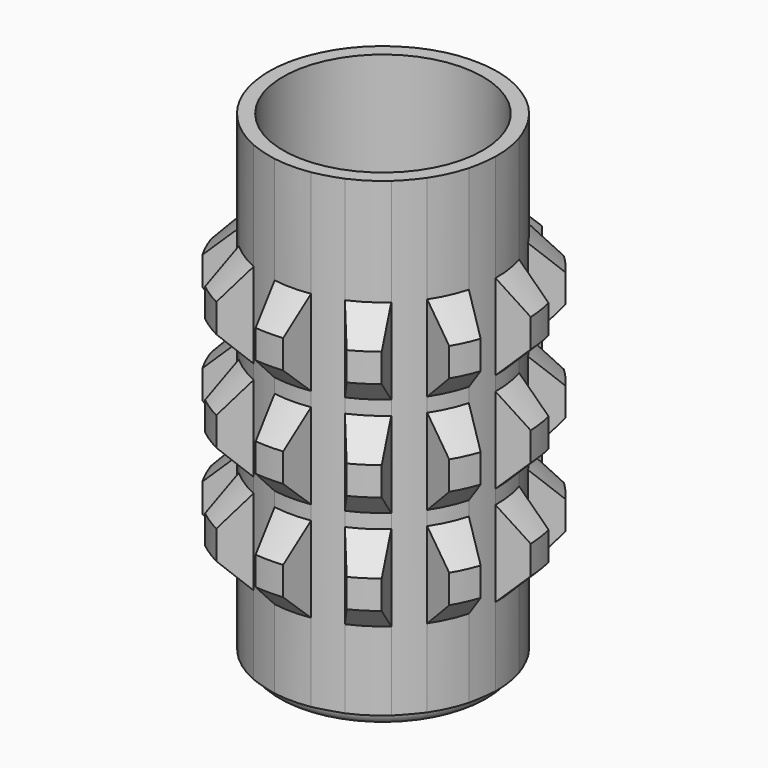
from build123d import *

# Parameters (mm, degrees)
F6_DEPTH = 225.001


# Not quite as in the source:
# - a feature names something its author has since deleted; it is built from what else it names


with BuildPart() as f1:
    # F0 (on Front) → F1 (revolve)
    with BuildSketch(Plane.XZ):
        with BuildLine():
            Line((40, -80), (40, 85))
            Line((40, 85), (35, 85))
            Line((35, 85), (35, -75))
            ThreePointArc((35, -75), (33.5355339059, -78.5355339059), (30, -80))
            Line((30, -80), (0, -80))
            Line((0, -80), (0, -85))
            Line((0, -85), (32.9289321881, -85))
            ThreePointArc((32.9289321881, -85), (37.5483298507, -81.9134171618), (36.4644660941, -76.4644660941))
            Line((36.4644660941, -76.4644660941), (40, -80))
        make_face()
    revolve(axis=Axis((0, 0, 2.5), (0, 0, 1)))

    # F2 (on Front) → F3 (revolve)
    with BuildSketch(Plane.XZ):
        Polygon((50, 37.5), (40, 47.5), (40, 17.5), (50, 27.5), align=None)
        Polygon((50, -7.5), (50, 2.5), (40, 12.5), (40, -17.5), align=None)
        Polygon((50, -42.5), (50, -32.5), (40, -22.5), (40, -52.5), align=None)
    revolve(axis=Axis((0, 0, 2.5), (0, 0, 1)))

    # F5 (on offset) → F6 (cut, through all)
    with BuildSketch(Plane.XY.offset(140)):
        with BuildLine():
            ThreePointArc((-18.8668219017, 48.0068175713), (-27.9042191508, 43.4198125328), (-35.8309761925, 37.104617598))
            Line((-35.8309761925, 37.104617598), (-25.6622849381, 30.6830104741))
            ThreePointArc((-25.6622849381, 30.6830104741), (-21.591517079, 33.5970563735), (-17.2497496098, 36.0894186487))
            Line((-17.2497496098, 36.0894186487), (-18.8668219017, 48.0068175713))
        make_face()
        with BuildLine():
            ThreePointArc((-5, 39.686269666), (0, 39.9368978106), (5, 39.686269666))
            Line((5, 39.686269666), (10.0826645171, 50.5860788976))
            ThreePointArc((10.0826645171, 50.5860788976), (0, 51.6132305402), (-10.0826645171, 50.5860788976))
            Line((-10.0826645171, 50.5860788976), (-5, 39.686269666))
        make_face()
        with BuildLine():
            ThreePointArc((-41.8262256733, 30.1857308662), (-46.949045883, 21.4409108359), (-50.2032060963, 11.8427023797))
            Line((-50.2032060963, 11.8427023797), (-38.1769757294, 11.9381122525))
            ThreePointArc((-38.1769757294, 11.9381122525), (-36.3278800438, 16.5903869233), (-34.0228255994, 21.0344322061))
            Line((-34.0228255994, 21.0344322061), (-41.8262256733, 30.1857308662))
        make_face()
        with BuildLine():
            ThreePointArc((-51.5060983236, 2.7808878932), (-51.0878822734, -7.3453285571), (-48.6362727834, -17.1791871675))
            Line((-48.6362727834, -17.1791871675), (-38.5707464723, -10.5970522586))
            ThreePointArc((-38.5707464723, -10.5970522586), (-39.5303977752, -5.6836131531), (-39.993894855, -0.6988378398))
            Line((-39.993894855, -0.6988378398), (-51.5060983236, 2.7808878932))
        make_face()
        with BuildLine():
            ThreePointArc((-44.8331486809, -25.5068673371), (-39.0066770118, -33.7994780328), (-31.6276665093, -40.7468061715))
            Line((-31.6276665093, -40.7468061715), (-26.718577738, -29.7677275528))
            ThreePointArc((-26.718577738, -29.7677275528), (-30.1822935214, -26.1531062118), (-33.2671850775, -22.2102318092))
            Line((-33.2671850775, -22.2102318092), (-44.8331486809, -25.5068673371))
        make_face()
        with BuildLine():
            ThreePointArc((-23.9259911079, -45.6963724108), (-14.5411274069, -49.5225320489), (-4.5774995889, -51.3776021191))
            Line((-4.5774995889, -51.3776021191), (-6.3834493564, -39.4873596777))
            ThreePointArc((-6.3834493564, -39.4873596777), (-11.2515243325, -38.3191728373), (-15.9783790926, -36.6700341093))
            Line((-15.9783790926, -36.6700341093), (-23.9259911079, -45.6963724108))
        make_face()
        with BuildLine():
            ThreePointArc((4.5774995889, -51.3776021191), (14.5411274069, -49.5225320489), (23.9259911079, -45.6963724108))
            Line((23.9259911079, -45.6963724108), (15.9783790926, -36.6700341093))
            ThreePointArc((15.9783790926, -36.6700341093), (11.2515243325, -38.3191728373), (6.3834493564, -39.4873596777))
            Line((6.3834493564, -39.4873596777), (4.5774995889, -51.3776021191))
        make_face()
        with BuildLine():
            ThreePointArc((31.6276665093, -40.7468061715), (39.0066770118, -33.7994780328), (44.8331486809, -25.5068673371))
            Line((44.8331486809, -25.5068673371), (33.2671850775, -22.2102318092))
            ThreePointArc((33.2671850775, -22.2102318092), (30.1822935214, -26.1531062118), (26.718577738, -29.7677275528))
            Line((26.718577738, -29.7677275528), (31.6276665093, -40.7468061715))
        make_face()
        with BuildLine():
            ThreePointArc((48.6362727834, -17.1791871675), (51.0878822734, -7.3453285571), (51.5060983236, 2.7808878932))
            Line((51.5060983236, 2.7808878932), (39.993894855, -0.6988378398))
            ThreePointArc((39.993894855, -0.6988378398), (39.5303977752, -5.6836131531), (38.5707464723, -10.5970522586))
            Line((38.5707464723, -10.5970522586), (48.6362727834, -17.1791871675))
        make_face()
        with BuildLine():
            ThreePointArc((50.2032060963, 11.8427023797), (46.949045883, 21.4409108359), (41.8262256733, 30.1857308662))
            Line((41.8262256733, 30.1857308662), (34.0228255994, 21.0344322061))
            ThreePointArc((34.0228255994, 21.0344322061), (36.3278800438, 16.5903869233), (38.1769757294, 11.9381122525))
            Line((38.1769757294, 11.9381122525), (50.2032060963, 11.8427023797))
        make_face()
        with BuildLine():
            ThreePointArc((35.8309761925, 37.104617598), (27.9042191508, 43.4198125328), (18.8668219017, 48.0068175713))
            Line((18.8668219017, 48.0068175713), (17.2497496098, 36.0894186487))
            ThreePointArc((17.2497496098, 36.0894186487), (21.591517079, 33.5970563735), (25.6622849381, 30.6830104741))
            Line((25.6622849381, 30.6830104741), (35.8309761925, 37.104617598))
        make_face()
    extrude(amount=-F6_DEPTH, mode=Mode.SUBTRACT)


solid = f1.part
